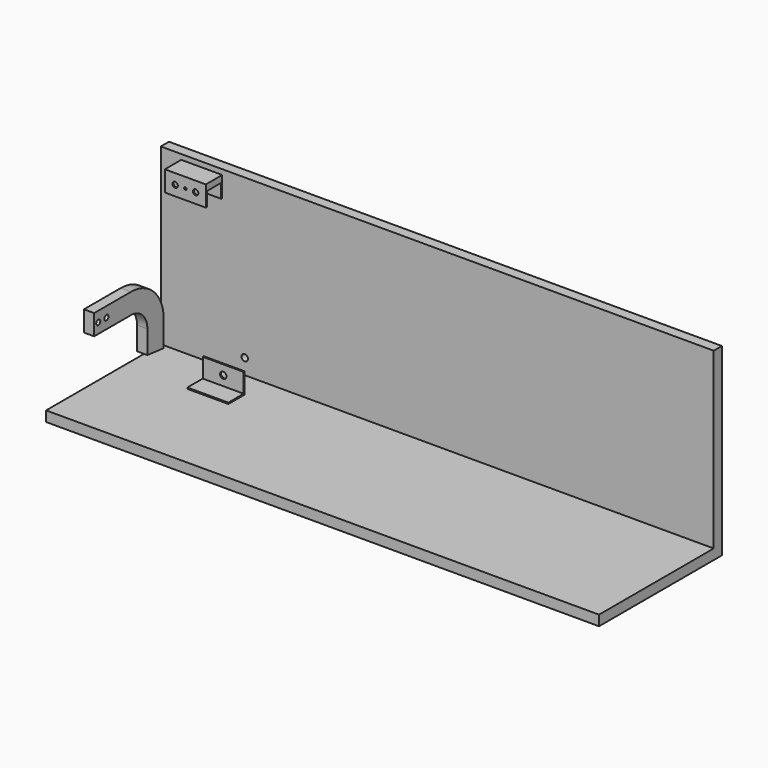
from build123d import *

# Parameters (mm, degrees)
F0_W      = 685.8
F0_H      = 215.9
F0_R      = 3.96875
F0_R_2    = 1.5875
F0_H_2    = 12.7
F1_DEPTH  = 12.7
F2_R      = 3.175
F3_DEPTH  = 12.7
F4_DEPTH  = 190.5
F5_W      = 50.8
F5_H      = 25.4
F6_DEPTH  = 1.5875
F7_W      = 50.8
F7_H      = 1.5875
F8_DEPTH  = 23.8125
F9_DEPTH  = 14.2885
F10_W     = 50.8
F10_H     = 25.4
F10_R     = 3.3734375
F10_R_2   = 1.5875
F11_DEPTH = 25.4
F12_W     = 22.225
F12_H     = 17.4625
F13_DEPTH = 660.401
F14_R     = 3.96875
F15_DEPTH = 46.0385


# Not quite as in the source:
# - a feature names something its author has since deleted; it is built from what else it names


with BuildPart() as f1:
    # F0 (on Front) → F1 (new body)
    with BuildSketch(Plane.XZ):
        with Locations((342.9, 107.95)):
            Rectangle(F0_W, F0_H)
        with Locations((104.14, 19.05)):
            Circle(F0_R, mode=Mode.SUBTRACT)
        with Locations((50.8, 196.85)):
            Circle(F0_R_2, mode=Mode.SUBTRACT)
        with Locations((342.9, -6.35)):
            Rectangle(F0_W, F0_H_2)
    extrude(amount=F1_DEPTH)

    # F0 (on Front) → F4 (join)
    with BuildSketch(Plane.XZ):
        with Locations((342.9, -6.35)):
            Rectangle(F0_W, F0_H_2)
    extrude(amount=F4_DEPTH)

    # F7 (on face) → F9 (cut, through all)
    with BuildSketch(Plane.XY.offset(1.5875)):
        with Locations((104.14, -45.24375)):
            Rectangle(F7_W, F7_H)
    extrude(amount=-F9_DEPTH, mode=Mode.SUBTRACT)


with BuildPart() as f3:
    # F2 (on Right) → F3 (new body)
    with BuildSketch(Plane.YZ):
        with BuildLine():
            Line((-131.8643205314, 86.509236245), (-131.8643205314, 61.109236245))
            Line((-131.8643205314, 61.109236245), (-74.7654969597, 61.109236245))
            ThreePointArc((-74.7654969597, 61.109236245), (-56.8049847175, 53.6697484872), (-49.3654969597, 35.709236245))
            Line((-49.3654969597, 35.709236245), (-49.3654969597, 7.134236245))
            Line((-49.3654969597, 7.134236245), (-23.9654969597, 4.357630532))
            Line((-23.9654969597, 4.357630532), (-23.9654969597, 35.709236245))
            ThreePointArc((-23.9654969597, 35.709236245), (-38.8444724754, 71.6302607293), (-74.7654969597, 86.509236245))
            Line((-74.7654969597, 86.509236245), (-131.8643205314, 86.509236245))
        make_face()
        with Locations((-125.5143205314, 73.809236245)):
            Circle(F2_R, mode=Mode.SUBTRACT)
        with Locations((-112.8143205314, 73.809236245)):
            Circle(F2_R, mode=Mode.SUBTRACT)
    extrude(amount=F3_DEPTH)


with BuildPart() as f6:
    # F5 (on face) → F6 (new body)
    with BuildSketch(Plane.XY):
        with Locations((104.14, -57.15)):
            Rectangle(F5_W, F5_H)
    extrude(amount=F6_DEPTH)

    # F7 (on face) → F8 (join)
    with BuildSketch(Plane.XY.offset(1.5875)):
        with Locations((104.14, -45.24375)):
            Rectangle(F7_W, F7_H)
    extrude(amount=F8_DEPTH)

    # F14 (on face) → F15 (cut, through all)
    with BuildSketch(Plane.XZ.offset(46.0375)):
        with Locations((104.14, 13.49375)):
            Circle(F14_R)
    extrude(amount=-F15_DEPTH, mode=Mode.SUBTRACT)


with BuildPart() as f11:
    # F10 (on face) → F11 (new body)
    with BuildSketch(Plane.XZ.offset(12.7)):
        with Locations((50.8, 196.85)):
            Rectangle(F10_W, F10_H)
        with Locations((38.1, 196.85)):
            Circle(F10_R, mode=Mode.SUBTRACT)
        with Locations((50.8, 196.85)):
            Circle(F10_R_2, mode=Mode.SUBTRACT)
        with Locations((63.5, 196.85)):
            Circle(F10_R, mode=Mode.SUBTRACT)
    extrude(amount=F11_DEPTH)

    # F12 (on face) → F13 (cut, through all)
    with BuildSketch(Plane(origin=(25.4, 0, 0), x_dir=(0, -1, 0), z_dir=(-1, 0, 0))):
        with Locations((25.4, 192.88125)):
            Rectangle(F12_W, F12_H)
    extrude(amount=-F13_DEPTH, mode=Mode.SUBTRACT)


solid = Compound([f1.part, f3.part, f6.part, f11.part])
